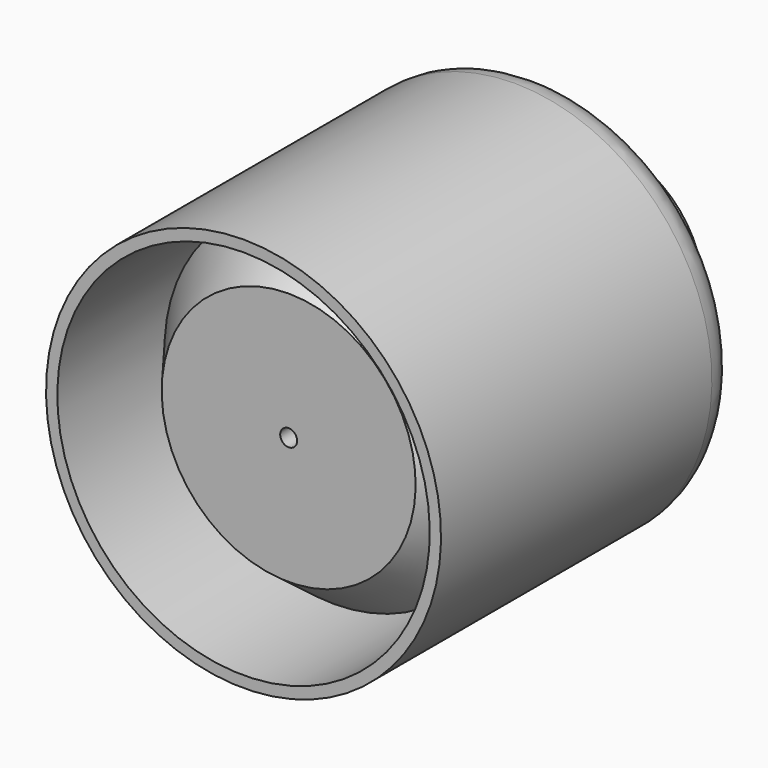
from build123d import *

# Parameters (mm, degrees)
F0_W     = 31.75
F0_H     = 76.2
F5_T     = -5.08
F3_R     = 3.81
F3_R_2   = 3.175
F7_DEPTH = 1270


# Not quite as in the source:
# - a feature of the source that left no trace in its solid (it failed there, or was rolled back) is left out


with BuildPart() as f1:
    # F0 (on Right) → F1 (revolve)
    with BuildSketch(Plane.YZ):
        with Locations((28.575, 38.1)):
            Rectangle(F0_W, F0_H)
    revolve(axis=Axis((0, 0, 0), (0, -1, 0)))


with BuildPart() as f1b:
    # F0 (on Right) → F1, piece 2 (revolve)
    with BuildSketch(Plane.YZ):
        Polygon((-76.2, 0), (-6.35, 0), (-6.35, 76.2), (-50.8, 76.2), (-76.2, 57.15), align=None)
    revolve(axis=Axis((0, 0, 0), (0, -1, 0)))


with BuildPart() as f4:
    # F0 (on Right) → F4 (revolve)
    with BuildSketch(Plane.YZ):
        with BuildLine():
            Line((44.45, 0), (101.6, 0))
            Line((101.6, 0), (101.6, 44.45))
            add(Edge.make_bspline(
                [(50.8, 88.9), (63.5, 88.9), (75.4157216212, 61.6914388631), (88.9, 44.45), (101.6, 44.45)],
                knots=[0, 0, 0, 0, 0.5154238597, 1, 1, 1, 1], degree=3))
            Line((50.8, 88.9), (-101.6, 88.9))
            Line((-101.6, 88.9), (-101.6, 0))
            Line((-101.6, 0), (-76.2, 0))
            Line((-76.2, 0), (-76.2, 57.15))
            Line((-76.2, 57.15), (-50.8, 76.2))
            Line((-50.8, 76.2), (-6.35, 76.2))
            Line((-6.35, 76.2), (-6.35, 0))
            Line((-6.35, 0), (12.7, 0))
            Line((12.7, 0), (12.7, 76.2))
            Line((12.7, 76.2), (44.45, 76.2))
            Line((44.45, 76.2), (44.45, 0))
        make_face()
        Polygon((-76.2, 0), (-6.35, 0), (-6.35, 76.2), (-50.8, 76.2), (-76.2, 57.15), align=None)
        with Locations((28.575, 38.1)):
            Rectangle(F0_W, F0_H)
    revolve(axis=Axis((0, 0, 0), (0, -1, 0)))

    # F5
    f5_openings = [f4.faces().sort_by_distance(p)[0] for p in [
        (0, -101.6, 0),
        (0, 101.6, 0),
    ]]
    offset(amount=F5_T, openings=f5_openings)


with BuildPart() as f7_tool:
    # F3 (on Front) → F7 (new body, symmetric)
    with BuildSketch(Plane.XZ):
        Circle(F3_R)
        Circle(F3_R_2, mode=Mode.SUBTRACT)
        Circle(F3_R_2)
    extrude(amount=F7_DEPTH, both=True)


with BuildPart() as f1_1:
    add(f1.part)

    # F7: cut by f7_tool
    add(f7_tool.part, mode=Mode.SUBTRACT)


with BuildPart() as f1b_1:
    add(f1b.part)

    # F7: cut by f7_tool
    add(f7_tool.part, mode=Mode.SUBTRACT)


solid = Compound([f4.part, f1_1.part, f1b_1.part])
